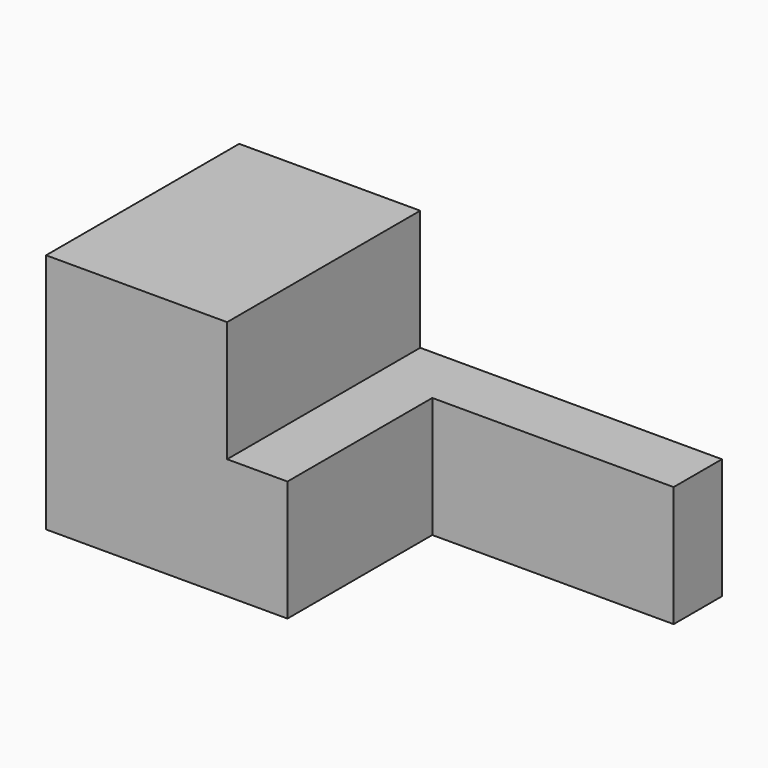
from build123d import *

# Parameters (mm, degrees)
F1_DEPTH = 101.6
F2_W     = 101.6
F2_H     = 76.2
F3_DEPTH = 50.8
F4_DEPTH = 50.8


# Not quite as in the source:
# - a feature names something its author has since deleted; it is built from what else it names


with BuildPart() as f1:
    # F0 (on Front) → F1 (new body)
    with BuildSketch(Plane.XZ):
        Polygon((0, 101.6), (0, 0), (203.2, 0), (203.2, 50.8), (76.2, 50.8), (76.2, 101.6), align=None)
    extrude(amount=F1_DEPTH)

    # F2 (on face) → F3 (cut)
    with BuildSketch(Plane.XY.offset(50.8)):
        with Locations((152.4, -63.5)):
            Rectangle(F2_W, F2_H)
    extrude(amount=-F3_DEPTH, mode=Mode.SUBTRACT)

    # F2 (on face) → F4 (cut)
    with BuildSketch(Plane.XY.offset(50.8)):
        with Locations((152.4, -63.5)):
            Rectangle(F2_W, F2_H)
    extrude(amount=-F4_DEPTH, mode=Mode.SUBTRACT)


solid = f1.part
